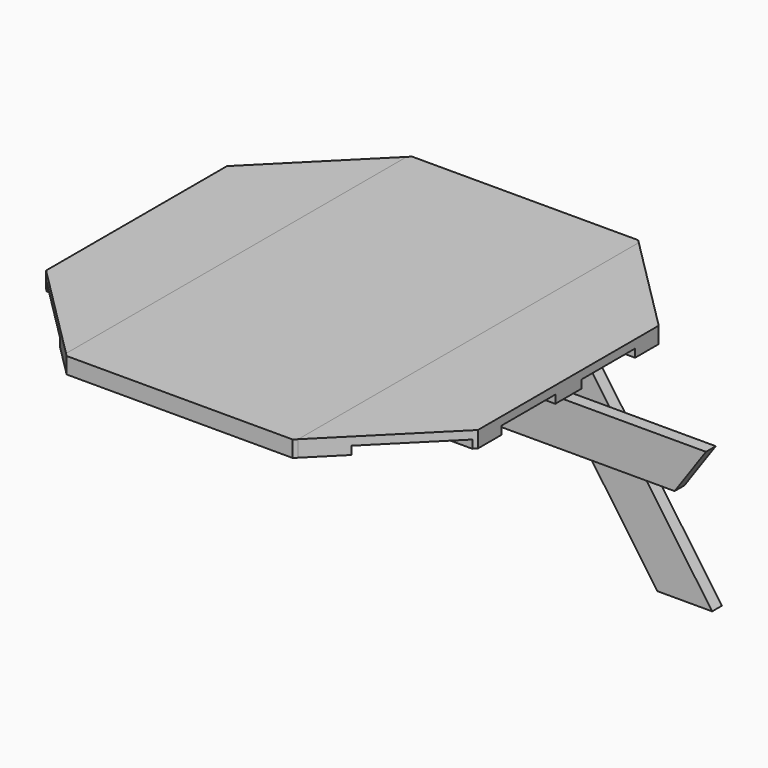
from build123d import *

# Parameters (mm, degrees)
F1_DEPTH  = 25.4
F0_W      = 311.15
F0_H      = 101.6
F0_H_2    = 209.55
F2_DEPTH  = 25.4
F3_DEPTH  = 25.4
F4_DEPTH  = 25.4
F5_DEPTH  = 25.4
F0_W_2    = 361.95
F6_DEPTH  = 25.4
F9_START  = 38.1
F9_DEPTH  = 38.1
F10_DEPTH = 38.1
F12_DEPTH = 69.85


with BuildPart() as f1:
    # F0 (on Top) → F1 (new body)
    with BuildSketch(Plane.XY):
        Polygon((-362.6062870026, 571.5), (-362.6062870026, 663.575), (-454.6812870026, 571.5), align=None)
    extrude(amount=-F1_DEPTH)



with BuildPart() as f1b:
    # F0 (on Top) → F1, piece 2 (new body)
    with BuildSketch(Plane.XY):
        Polygon((-362.6062870026, 260.35), (-362.6062870026, 361.95), (-664.2312870026, 361.95), (-673.7562870026, 352.425), (-673.7562870026, 260.35), align=None)
    extrude(amount=-F1_DEPTH)


with BuildPart() as f1c:
    # F0 (on Top) → F1, piece 3 (new body)
    with BuildSketch(Plane.XY):
        with Locations((-518.1812870026, 0)):
            Rectangle(F0_W, F0_H)
    extrude(amount=-F1_DEPTH)


with BuildPart() as f1d:
    # F0 (on Top) → F1, piece 4 (new body)
    with BuildSketch(Plane.XY):
        Polygon((-362.6062870026, -361.95), (-362.6062870026, -260.35), (-673.7562870026, -260.35), (-673.7562870026, -352.425), (-664.2312870026, -361.95), align=None)
    extrude(amount=-F1_DEPTH)


with BuildPart() as f1e:
    # F0 (on Top) → F1, piece 5 (new body)
    with BuildSketch(Plane.XY):
        Polygon((-362.6062870026, -663.575), (-362.6062870026, -571.5), (-454.6812870026, -571.5), align=None)
    extrude(amount=-F1_DEPTH)


with BuildPart() as f1_1:
    add(f1.part)

    add(f1b.part)  # F2 merges F1b

    add(f1c.part)  # F2 merges F1c

    add(f1d.part)  # F2 merges F1d

    add(f1e.part)  # F2 merges F1e
    # F0 (on Top) → F2 (join)
    with BuildSketch(Plane.XY):
        Polygon((-362.6062870026, 571.5), (-362.6062870026, 663.575), (-454.6812870026, 571.5), align=None)
        Polygon((-362.6062870026, 361.95), (-362.6062870026, 571.5), (-454.6812870026, 571.5), (-664.2312870026, 361.95), align=None)
        Polygon((-362.6062870026, 260.35), (-362.6062870026, 361.95), (-664.2312870026, 361.95), (-673.7562870026, 352.425), (-673.7562870026, 260.35), align=None)
        with Locations((-518.1812870026, 155.575)):
            Rectangle(F0_W, F0_H_2)
        with Locations((-518.1812870026, 0)):
            Rectangle(F0_W, F0_H)
        with Locations((-518.1812870026, -155.575)):
            Rectangle(F0_W, F0_H_2)
        Polygon((-362.6062870026, -361.95), (-362.6062870026, -260.35), (-673.7562870026, -260.35), (-673.7562870026, -352.425), (-664.2312870026, -361.95), align=None)
        Polygon((-362.6062870026, -571.5), (-362.6062870026, -361.95), (-664.2312870026, -361.95), (-454.6812870026, -571.5), align=None)
        Polygon((-362.6062870026, -663.575), (-362.6062870026, -571.5), (-454.6812870026, -571.5), align=None)
    extrude(amount=F2_DEPTH)


with BuildPart() as f3:
    # F0 (on Top) → F3 (new body)
    with BuildSketch(Plane.XY):
        Polygon((361.2937129974, 663.575), (361.2937129974, 571.5), (453.3687129974, 571.5), align=None)
    extrude(amount=-F3_DEPTH)



with BuildPart() as f3b:
    # F0 (on Top) → F3, piece 2 (new body)
    with BuildSketch(Plane.XY):
        Polygon((662.9187129974, 361.95), (361.2937129974, 361.95), (361.2937129974, 260.35), (672.4437129974, 260.35), (672.4437129974, 352.425), align=None)
    extrude(amount=-F3_DEPTH)


with BuildPart() as f3c:
    # F0 (on Top) → F3, piece 3 (new body)
    with BuildSketch(Plane.XY):
        with Locations((516.8687129974, 0)):
            Rectangle(F0_W, F0_H)
    extrude(amount=-F3_DEPTH)


with BuildPart() as f3d:
    # F0 (on Top) → F3, piece 4 (new body)
    with BuildSketch(Plane.XY):
        Polygon((672.4437129974, -260.35), (361.2937129974, -260.35), (361.2937129974, -361.95), (662.9187129974, -361.95), (672.4437129974, -352.425), align=None)
    extrude(amount=-F3_DEPTH)


with BuildPart() as f3e:
    # F0 (on Top) → F3, piece 5 (new body)
    with BuildSketch(Plane.XY):
        Polygon((453.3687129974, -571.5), (361.2937129974, -571.5), (361.2937129974, -663.575), align=None)
    extrude(amount=-F3_DEPTH)


with BuildPart() as f3_1:
    add(f3.part)

    add(f3b.part)  # F4 merges F3b

    add(f3c.part)  # F4 merges F3c

    add(f3d.part)  # F4 merges F3d

    add(f3e.part)  # F4 merges F3e
    # F0 (on Top) → F4 (join)
    with BuildSketch(Plane.XY):
        Polygon((361.2937129974, 663.575), (361.2937129974, 571.5), (453.3687129974, 571.5), align=None)
        Polygon((453.3687129974, 571.5), (361.2937129974, 571.5), (361.2937129974, 361.95), (662.9187129974, 361.95), align=None)
        Polygon((662.9187129974, 361.95), (361.2937129974, 361.95), (361.2937129974, 260.35), (672.4437129974, 260.35), (672.4437129974, 352.425), align=None)
        with Locations((516.8687129974, 155.575)):
            Rectangle(F0_W, F0_H_2)
        with Locations((516.8687129974, 0)):
            Rectangle(F0_W, F0_H)
        with Locations((516.8687129974, -155.575)):
            Rectangle(F0_W, F0_H_2)
        Polygon((672.4437129974, -260.35), (361.2937129974, -260.35), (361.2937129974, -361.95), (662.9187129974, -361.95), (672.4437129974, -352.425), align=None)
        Polygon((662.9187129974, -361.95), (361.2937129974, -361.95), (361.2937129974, -571.5), (453.3687129974, -571.5), align=None)
        Polygon((453.3687129974, -571.5), (361.2937129974, -571.5), (361.2937129974, -663.575), align=None)
    extrude(amount=F4_DEPTH)


with BuildPart() as f5:
    # F0 (on Top) → F5 (new body)
    with BuildSketch(Plane.XY):
        Polygon((-353.0812870026, 673.1), (-362.6062870026, 663.575), (-362.6062870026, 571.5), (-0.6562870026, 571.5), (-0.6562870026, 673.1), align=None)
        Polygon((-0.6562870026, 673.1), (-0.6562870026, 571.5), (361.2937129974, 571.5), (361.2937129974, 663.575), (351.7687129974, 673.1), align=None)
    extrude(amount=-F5_DEPTH)



with BuildPart() as f5b:
    # F0 (on Top) → F5, piece 2 (new body)
    with BuildSketch(Plane.XY):
        with Locations((-181.6312870026, 311.15)):
            Rectangle(F0_W_2, F0_H)
        with Locations((180.3187129974, 311.15)):
            Rectangle(F0_W_2, F0_H)
    extrude(amount=-F5_DEPTH)


with BuildPart() as f5c:
    # F0 (on Top) → F5, piece 3 (new body)
    with BuildSketch(Plane.XY):
        with Locations((-181.6312870026, 0)):
            Rectangle(F0_W_2, F0_H)
        with Locations((180.3187129974, 0)):
            Rectangle(F0_W_2, F0_H)
    extrude(amount=-F5_DEPTH)


with BuildPart() as f5d:
    # F0 (on Top) → F5, piece 4 (new body)
    with BuildSketch(Plane.XY):
        with Locations((-181.6312870026, -311.15)):
            Rectangle(F0_W_2, F0_H)
        with Locations((180.3187129974, -311.15)):
            Rectangle(F0_W_2, F0_H)
    extrude(amount=-F5_DEPTH)


with BuildPart() as f5e:
    # F0 (on Top) → F5, piece 5 (new body)
    with BuildSketch(Plane.XY):
        Polygon((-0.6562870026, -571.5), (-362.6062870026, -571.5), (-362.6062870026, -663.575), (-353.0812870026, -673.1), (-0.6562870026, -673.1), align=None)
        Polygon((361.2937129974, -571.5), (-0.6562870026, -571.5), (-0.6562870026, -673.1), (351.7687129974, -673.1), (361.2937129974, -663.575), align=None)
    extrude(amount=-F5_DEPTH)


with BuildPart() as f5_1:
    add(f5.part)

    add(f5b.part)  # F6 merges F5b

    add(f5c.part)  # F6 merges F5c

    add(f5d.part)  # F6 merges F5d

    add(f5e.part)  # F6 merges F5e
    # F0 (on Top) → F6 (join)
    with BuildSketch(Plane.XY):
        with Locations((-181.6312870026, 466.725)):
            Rectangle(F0_W_2, F0_H_2)
        with Locations((180.3187129974, 466.725)):
            Rectangle(F0_W_2, F0_H_2)
        Polygon((-353.0812870026, 673.1), (-362.6062870026, 663.575), (-362.6062870026, 571.5), (-0.6562870026, 571.5), (-0.6562870026, 673.1), align=None)
        Polygon((-0.6562870026, 673.1), (-0.6562870026, 571.5), (361.2937129974, 571.5), (361.2937129974, 663.575), (351.7687129974, 673.1), align=None)
        with Locations((-181.6312870026, 311.15)):
            Rectangle(F0_W_2, F0_H)
        with Locations((180.3187129974, 311.15)):
            Rectangle(F0_W_2, F0_H)
        with Locations((-181.6312870026, 155.575)):
            Rectangle(F0_W_2, F0_H_2)
        with Locations((180.3187129974, 155.575)):
            Rectangle(F0_W_2, F0_H_2)
        with Locations((180.3187129974, 0)):
            Rectangle(F0_W_2, F0_H)
        with Locations((-181.6312870026, 0)):
            Rectangle(F0_W_2, F0_H)
        with Locations((-181.6312870026, -155.575)):
            Rectangle(F0_W_2, F0_H_2)
        with Locations((180.3187129974, -155.575)):
            Rectangle(F0_W_2, F0_H_2)
        with Locations((180.3187129974, -311.15)):
            Rectangle(F0_W_2, F0_H)
        with Locations((-181.6312870026, -311.15)):
            Rectangle(F0_W_2, F0_H)
        with Locations((-181.6312870026, -466.725)):
            Rectangle(F0_W_2, F0_H_2)
        with Locations((180.3187129974, -466.725)):
            Rectangle(F0_W_2, F0_H_2)
        Polygon((361.2937129974, -571.5), (-0.6562870026, -571.5), (-0.6562870026, -673.1), (351.7687129974, -673.1), (361.2937129974, -663.575), align=None)
        Polygon((-0.6562870026, -571.5), (-362.6062870026, -571.5), (-362.6062870026, -663.575), (-353.0812870026, -673.1), (-0.6562870026, -673.1), align=None)
    extrude(amount=F6_DEPTH)


with BuildPart() as f9:
    # F8 (on line) → F9 (new body)
    with BuildSketch(Plane(origin=(0, 361.95, 0), x_dir=(-1, 0, 0), z_dir=(0, 1, 0)).offset(F9_START)):
        Polygon((-212.3704960354, -139.7), (-114.5515029475, 0), (-285.0937129974, 0), (-323.1937129974, -54.4124390569), (-263.4747199095, -139.7), align=None)
        Polygon((-310.1894891233, -279.4), (-212.3704960354, -139.7), (-263.4747199095, -139.7), (-323.1937129974, -54.4124390569), (-480.7316991732, -279.4), align=None)
        Polygon((-408.0084822112, -419.1), (-310.1894891233, -279.4), (-480.7316991732, -279.4), (-578.5506922611, -419.1), align=None)
        Polygon((-630.3243755927, -736.6), (-408.0084822112, -419.1), (-578.5506922611, -419.1), (-800.8665856427, -736.6), align=None)
    extrude(amount=F9_DEPTH)


with BuildPart() as f9b:
    # F8 (on line) → F9, piece 2 (new body)
    with BuildSketch(Plane(origin=(0, 361.95, 0), x_dir=(-1, 0, 0), z_dir=(0, 1, 0)).offset(F9_START)):
        Polygon((579.8632662663, -419.1), (409.3210562163, -419.1), (631.6369495979, -736.6), (802.1791596478, -736.6), align=None)
        Polygon((482.0442731784, -279.4), (311.5020631284, -279.4), (409.3210562163, -419.1), (579.8632662663, -419.1), align=None)
        Polygon((264.7872939147, -139.7), (213.6830700405, -139.7), (311.5020631284, -279.4), (482.0442731784, -279.4), (324.5062870026, -54.4124390569), align=None)
        Polygon((286.4062870026, 0), (115.8640769526, 0), (213.6830700405, -139.7), (264.7872939147, -139.7), (324.5062870026, -54.4124390569), align=None)
    extrude(amount=F9_DEPTH)


with BuildPart() as f10:
    # F8 (on line) → F10 (new body)
    with BuildSketch(Plane(origin=(0, 361.95, 0), x_dir=(-1, 0, 0), z_dir=(0, 1, 0))):
        Polygon((-212.3704960354, -139.7), (-114.5515029475, 0), (-285.0937129974, 0), (-323.1937129974, -54.4124390569), (-263.4747199095, -139.7), align=None)
        Polygon((0.6562870026, -139.7), (0.6562870026, 0), (-114.5515029475, 0), (-212.3704960354, -139.7), align=None)
        Polygon((115.8640769526, 0), (0.6562870026, 0), (0.6562870026, -139.7), (213.6830700405, -139.7), align=None)
        Polygon((286.4062870026, 0), (115.8640769526, 0), (213.6830700405, -139.7), (264.7872939147, -139.7), (324.5062870026, -54.4124390569), align=None)
        Polygon((-323.1937129974, -54.4124390569), (-285.0937129974, 0), (-361.2937129974, 0), align=None)
        Polygon((362.6062870026, 0), (286.4062870026, 0), (324.5062870026, -54.4124390569), align=None)
    extrude(amount=F10_DEPTH)


with BuildPart() as f10b:
    # F8 (on line) → F10, piece 2 (new body)
    with BuildSketch(Plane(origin=(0, 361.95, 0), x_dir=(-1, 0, 0), z_dir=(0, 1, 0))):
        Polygon((0.6562870026, -279.4), (-310.1894891233, -279.4), (-408.0084822112, -419.1), (0.6562870026, -419.1), align=None)
        Polygon((409.3210562163, -419.1), (311.5020631284, -279.4), (0.6562870026, -279.4), (0.6562870026, -419.1), align=None)
        Polygon((482.0442731784, -279.4), (311.5020631284, -279.4), (409.3210562163, -419.1), (579.8632662663, -419.1), align=None)
        Polygon((813.4562870026, -279.4), (482.0442731784, -279.4), (579.8632662663, -419.1), (715.6372939147, -419.1), align=None)
        Polygon((-408.0084822112, -419.1), (-310.1894891233, -279.4), (-480.7316991732, -279.4), (-578.5506922611, -419.1), align=None)
        Polygon((-578.5506922611, -419.1), (-480.7316991732, -279.4), (-812.1437129974, -279.4), (-714.3247199095, -419.1), align=None)
    extrude(amount=F10_DEPTH)


with BuildPart() as f12:
    # F11 (on Right) → F12 (new body, symmetric)
    with BuildSketch(Plane.YZ):
        Polygon((406.2173252089, -279.4), (571.5, 0), (546.7129550388, 0), (527.2326747911, 0), (361.95, -279.4), align=None)
    extrude(amount=F12_DEPTH, both=True)


solid = Compound([f1_1.part, f3_1.part, f5_1.part, f9.part, f9b.part, f10.part, f10b.part, f12.part])
